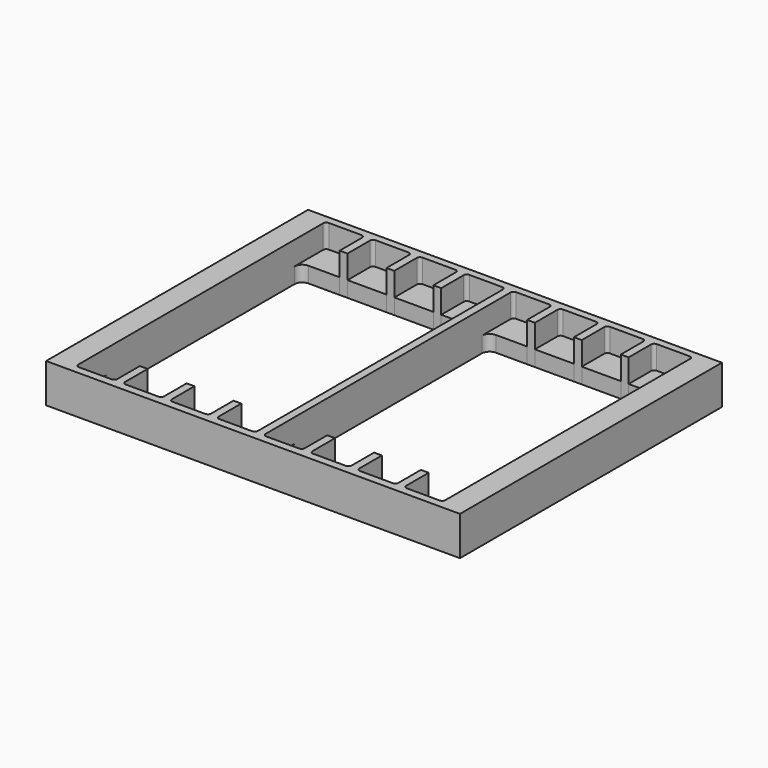
from build123d import *

# Parameters (mm, degrees)
F3_DEPTH = 10
F4_DEPTH = 10
F6_DEPTH = 25
F7_DEPTH = 25
F8_DEPTH = 25


# Not quite as in the source:
# - a feature names something its author has since deleted; it is built from what else it names


with BuildPart() as f3:
    # F0 (on Top) → F3 (new body)
    with BuildSketch(Plane.XY):
        Polygon((0, 104.6779751778), (-132.5, 104.6779751778), (-132.5, -105), (0, -105), (132.5, -105), (132.5, 104.6779751778), align=None)
        with BuildLine():
            Line((-57.5, -80), (-62.5, -80))
            Line((-62.5, -80), (-62.5, -98))
            ThreePointArc((-62.5, -98), (-63.0857864376, -99.4142135624), (-64.5, -100))
            Line((-64.5, -100), (-85.5, -100))
            ThreePointArc((-85.5, -100), (-86.9142135624, -99.4142135624), (-87.5, -98))
            Line((-87.5, -98), (-87.5, -80))
            Line((-87.5, -80), (-92.5, -80))
            Line((-92.5, -80), (-92.5, -98))
            ThreePointArc((-92.5, -98), (-93.0857864376, -99.4142135624), (-94.5, -100))
            Line((-94.5, -100), (-115.5, -100))
            ThreePointArc((-115.5, -100), (-116.9142135624, -99.4142135624), (-117.5, -98))
            Line((-117.5, -98), (-117.5, -75))
            Line((-117.5, -75), (-117.5, 75))
            Line((-117.5, 75), (-117.5, 98))
            ThreePointArc((-117.5, 98), (-116.9142135624, 99.4142135624), (-115.5, 100))
            Line((-115.5, 100), (-94.5, 100))
            ThreePointArc((-94.5, 100), (-93.0857864376, 99.4142135624), (-92.5, 98))
            Line((-92.5, 98), (-92.5, 80))
            Line((-92.5, 80), (-87.5, 80))
            Line((-87.5, 80), (-87.5, 98))
            ThreePointArc((-87.5, 98), (-86.9142135624, 99.4142135624), (-85.5, 100))
            Line((-85.5, 100), (-64.5, 100))
            ThreePointArc((-64.5, 100), (-63.0857864376, 99.4142135624), (-62.5, 98))
            Line((-62.5, 98), (-62.5, 80))
            Line((-62.5, 80), (-57.5, 80))
            Line((-57.5, 80), (-57.5, 98))
            ThreePointArc((-57.5, 98), (-56.9142135624, 99.4142135624), (-55.5, 100))
            Line((-55.5, 100), (-34.5, 100))
            ThreePointArc((-34.5, 100), (-33.0857864376, 99.4142135624), (-32.5, 98))
            Line((-32.5, 98), (-32.5, 80))
            Line((-32.5, 80), (-27.5, 80))
            Line((-27.5, 80), (-27.5, 98))
            ThreePointArc((-27.5, 98), (-26.9142135624, 99.4142135624), (-25.5, 100))
            Line((-25.5, 100), (-4.5, 100))
            ThreePointArc((-4.5, 100), (-3.0857864376, 99.4142135624), (-2.5, 98))
            Line((-2.5, 98), (-2.5, 75))
            Line((-2.5, 75), (-2.5, -75))
            Line((-2.5, -75), (-2.5, -98))
            ThreePointArc((-2.5, -98), (-3.0857864376, -99.4142135624), (-4.5, -100))
            Line((-4.5, -100), (-25.5, -100))
            ThreePointArc((-25.5, -100), (-26.9142135624, -99.4142135624), (-27.5, -98))
            Line((-27.5, -98), (-27.5, -80))
            Line((-27.5, -80), (-32.5, -80))
            Line((-32.5, -80), (-32.5, -98))
            ThreePointArc((-32.5, -98), (-33.0857864376, -99.4142135624), (-34.5, -100))
            Line((-34.5, -100), (-55.5, -100))
            ThreePointArc((-55.5, -100), (-56.9142135624, -99.4142135624), (-57.5, -98))
            Line((-57.5, -98), (-57.5, -80))
        make_face(mode=Mode.SUBTRACT)
        with BuildLine():
            Line((92.5, 80), (92.5, 98))
            ThreePointArc((92.5, 98), (93.0857864376, 99.4142135624), (94.5, 100))
            Line((94.5, 100), (115.5, 100))
            ThreePointArc((115.5, 100), (116.9142135624, 99.4142135624), (117.5, 98))
            Line((117.5, 98), (117.5, 75))
            Line((117.5, 75), (117.5, -75))
            Line((117.5, -75), (117.5, -98))
            ThreePointArc((117.5, -98), (116.9142135624, -99.4142135624), (115.5, -100))
            Line((115.5, -100), (94.5, -100))
            ThreePointArc((94.5, -100), (93.0857864376, -99.4142135624), (92.5, -98))
            Line((92.5, -98), (92.5, -80))
            Line((92.5, -80), (87.5, -80))
            Line((87.5, -80), (87.5, -98))
            ThreePointArc((87.5, -98), (86.9142135624, -99.4142135624), (85.5, -100))
            Line((85.5, -100), (64.5, -100))
            ThreePointArc((64.5, -100), (63.0857864376, -99.4142135624), (62.5, -98))
            Line((62.5, -98), (62.5, -80))
            Line((62.5, -80), (57.5, -80))
            Line((57.5, -80), (57.5, -98))
            ThreePointArc((57.5, -98), (56.9142135624, -99.4142135624), (55.5, -100))
            Line((55.5, -100), (34.5, -100))
            ThreePointArc((34.5, -100), (33.0857864376, -99.4142135624), (32.5, -98))
            Line((32.5, -98), (32.5, -80))
            Line((32.5, -80), (27.5, -80))
            Line((27.5, -80), (27.5, -98))
            ThreePointArc((27.5, -98), (26.9142135624, -99.4142135624), (25.5, -100))
            Line((25.5, -100), (4.5, -100))
            ThreePointArc((4.5, -100), (3.0857864376, -99.4142135624), (2.5, -98))
            Line((2.5, -98), (2.5, -75))
            Line((2.5, -75), (2.5, 75))
            Line((2.5, 75), (2.5, 98))
            ThreePointArc((2.5, 98), (3.0857864376, 99.4142135624), (4.5, 100))
            Line((4.5, 100), (25.5, 100))
            ThreePointArc((25.5, 100), (26.9142135624, 99.4142135624), (27.5, 98))
            Line((27.5, 98), (27.5, 80))
            Line((27.5, 80), (32.5, 80))
            Line((32.5, 80), (32.5, 98))
            ThreePointArc((32.5, 98), (33.0857864376, 99.4142135624), (34.5, 100))
            Line((34.5, 100), (55.5, 100))
            ThreePointArc((55.5, 100), (56.9142135624, 99.4142135624), (57.5, 98))
            Line((57.5, 98), (57.5, 80))
            Line((57.5, 80), (62.5, 80))
            Line((62.5, 80), (62.5, 98))
            ThreePointArc((62.5, 98), (63.0857864376, 99.4142135624), (64.5, 100))
            Line((64.5, 100), (85.5, 100))
            ThreePointArc((85.5, 100), (86.9142135624, 99.4142135624), (87.5, 98))
            Line((87.5, 98), (87.5, 80))
            Line((87.5, 80), (92.5, 80))
        make_face(mode=Mode.SUBTRACT)
        with BuildLine():
            ThreePointArc((-7.5, 80), (-3.9644660941, 78.5355339059), (-2.5, 75))
            Line((-2.5, 75), (-2.5, 98))
            ThreePointArc((-2.5, 98), (-3.0857864376, 99.4142135624), (-4.5, 100))
            Line((-4.5, 100), (-25.5, 100))
            ThreePointArc((-25.5, 100), (-26.9142135624, 99.4142135624), (-27.5, 98))
            Line((-27.5, 98), (-27.5, 80))
            Line((-27.5, 80), (-7.5, 80))
        make_face()
        with BuildLine():
            Line((-92.5, -98), (-92.5, -80))
            Line((-92.5, -80), (-112.5, -80))
            ThreePointArc((-112.5, -80), (-116.0355339059, -78.5355339059), (-117.5, -75))
            Line((-117.5, -75), (-117.5, -98))
            ThreePointArc((-117.5, -98), (-116.9142135624, -99.4142135624), (-115.5, -100))
            Line((-115.5, -100), (-94.5, -100))
            ThreePointArc((-94.5, -100), (-93.0857864376, -99.4142135624), (-92.5, -98))
        make_face()
        with BuildLine():
            Line((-7.5, -80), (-27.5, -80))
            Line((-27.5, -80), (-27.5, -98))
            ThreePointArc((-27.5, -98), (-26.9142135624, -99.4142135624), (-25.5, -100))
            Line((-25.5, -100), (-4.5, -100))
            ThreePointArc((-4.5, -100), (-3.0857864376, -99.4142135624), (-2.5, -98))
            Line((-2.5, -98), (-2.5, -75))
            ThreePointArc((-2.5, -75), (-3.9644660941, -78.5355339059), (-7.5, -80))
        make_face()
        with BuildLine():
            Line((-117.5, 98), (-117.5, 75))
            ThreePointArc((-117.5, 75), (-116.0355339059, 78.5355339059), (-112.5, 80))
            Line((-112.5, 80), (-92.5, 80))
            Line((-92.5, 80), (-92.5, 98))
            ThreePointArc((-92.5, 98), (-93.0857864376, 99.4142135624), (-94.5, 100))
            Line((-94.5, 100), (-115.5, 100))
            ThreePointArc((-115.5, 100), (-116.9142135624, 99.4142135624), (-117.5, 98))
        make_face()
        with BuildLine():
            Line((-87.5, 98), (-87.5, 80))
            Line((-87.5, 80), (-62.5, 80))
            Line((-62.5, 80), (-62.5, 98))
            ThreePointArc((-62.5, 98), (-63.0857864376, 99.4142135624), (-64.5, 100))
            Line((-64.5, 100), (-85.5, 100))
            ThreePointArc((-85.5, 100), (-86.9142135624, 99.4142135624), (-87.5, 98))
        make_face()
        with BuildLine():
            Line((-57.5, 80), (-32.5, 80))
            Line((-32.5, 80), (-32.5, 98))
            ThreePointArc((-32.5, 98), (-33.0857864376, 99.4142135624), (-34.5, 100))
            Line((-34.5, 100), (-55.5, 100))
            ThreePointArc((-55.5, 100), (-56.9142135624, 99.4142135624), (-57.5, 98))
            Line((-57.5, 98), (-57.5, 80))
        make_face()
        with BuildLine():
            Line((-62.5, -98), (-62.5, -80))
            Line((-62.5, -80), (-87.5, -80))
            Line((-87.5, -80), (-87.5, -98))
            ThreePointArc((-87.5, -98), (-86.9142135624, -99.4142135624), (-85.5, -100))
            Line((-85.5, -100), (-64.5, -100))
            ThreePointArc((-64.5, -100), (-63.0857864376, -99.4142135624), (-62.5, -98))
        make_face()
        with BuildLine():
            Line((-32.5, -80), (-57.5, -80))
            Line((-57.5, -80), (-57.5, -98))
            ThreePointArc((-57.5, -98), (-56.9142135624, -99.4142135624), (-55.5, -100))
            Line((-55.5, -100), (-34.5, -100))
            ThreePointArc((-34.5, -100), (-33.0857864376, -99.4142135624), (-32.5, -98))
            Line((-32.5, -98), (-32.5, -80))
        make_face()
    extrude(amount=F3_DEPTH)

    # F0 (on Top) → F4 (join)
    with BuildSketch(Plane.XY):
        with BuildLine():
            Line((7.5, 80), (27.5, 80))
            Line((27.5, 80), (27.5, 98))
            ThreePointArc((27.5, 98), (26.9142135624, 99.4142135624), (25.5, 100))
            Line((25.5, 100), (4.5, 100))
            ThreePointArc((4.5, 100), (3.0857864376, 99.4142135624), (2.5, 98))
            Line((2.5, 98), (2.5, 75))
            ThreePointArc((2.5, 75), (3.9644660941, 78.5355339059), (7.5, 80))
        make_face()
        with BuildLine():
            Line((32.5, 80), (57.5, 80))
            Line((57.5, 80), (57.5, 98))
            ThreePointArc((57.5, 98), (56.9142135624, 99.4142135624), (55.5, 100))
            Line((55.5, 100), (34.5, 100))
            ThreePointArc((34.5, 100), (33.0857864376, 99.4142135624), (32.5, 98))
            Line((32.5, 98), (32.5, 80))
        make_face()
        with BuildLine():
            Line((62.5, 80), (87.5, 80))
            Line((87.5, 80), (87.5, 98))
            ThreePointArc((87.5, 98), (86.9142135624, 99.4142135624), (85.5, 100))
            Line((85.5, 100), (64.5, 100))
            ThreePointArc((64.5, 100), (63.0857864376, 99.4142135624), (62.5, 98))
            Line((62.5, 98), (62.5, 80))
        make_face()
        with BuildLine():
            ThreePointArc((94.5, 100), (93.0857864376, 99.4142135624), (92.5, 98))
            Line((92.5, 98), (92.5, 80))
            Line((92.5, 80), (112.5, 80))
            ThreePointArc((112.5, 80), (116.0355339059, 78.5355339059), (117.5, 75))
            Line((117.5, 75), (117.5, 98))
            ThreePointArc((117.5, 98), (116.9142135624, 99.4142135624), (115.5, 100))
            Line((115.5, 100), (94.5, 100))
        make_face()
        with BuildLine():
            Line((117.5, -98), (117.5, -75))
            ThreePointArc((117.5, -75), (116.0355339059, -78.5355339059), (112.5, -80))
            Line((112.5, -80), (92.5, -80))
            Line((92.5, -80), (92.5, -98))
            ThreePointArc((92.5, -98), (93.0857864376, -99.4142135624), (94.5, -100))
            Line((94.5, -100), (115.5, -100))
            ThreePointArc((115.5, -100), (116.9142135624, -99.4142135624), (117.5, -98))
        make_face()
        with BuildLine():
            Line((87.5, -98), (87.5, -80))
            Line((87.5, -80), (62.5, -80))
            Line((62.5, -80), (62.5, -98))
            ThreePointArc((62.5, -98), (63.0857864376, -99.4142135624), (64.5, -100))
            Line((64.5, -100), (85.5, -100))
            ThreePointArc((85.5, -100), (86.9142135624, -99.4142135624), (87.5, -98))
        make_face()
        with BuildLine():
            Line((57.5, -98), (57.5, -80))
            Line((57.5, -80), (32.5, -80))
            Line((32.5, -80), (32.5, -98))
            ThreePointArc((32.5, -98), (33.0857864376, -99.4142135624), (34.5, -100))
            Line((34.5, -100), (55.5, -100))
            ThreePointArc((55.5, -100), (56.9142135624, -99.4142135624), (57.5, -98))
        make_face()
        with BuildLine():
            ThreePointArc((7.5, -80), (3.9644660941, -78.5355339059), (2.5, -75))
            Line((2.5, -75), (2.5, -98))
            ThreePointArc((2.5, -98), (3.0857864376, -99.4142135624), (4.5, -100))
            Line((4.5, -100), (25.5, -100))
            ThreePointArc((25.5, -100), (26.9142135624, -99.4142135624), (27.5, -98))
            Line((27.5, -98), (27.5, -80))
            Line((27.5, -80), (7.5, -80))
        make_face()
    extrude(amount=F4_DEPTH)


with BuildPart() as f6:
    # F0 (on Top) → F6 (new body)
    with BuildSketch(Plane.XY):
        Polygon((0, 104.6779751778), (-132.5, 104.6779751778), (-132.5, -105), (0, -105), (132.5, -105), (132.5, 104.6779751778), align=None)
        with BuildLine():
            Line((-57.5, -80), (-62.5, -80))
            Line((-62.5, -80), (-62.5, -98))
            ThreePointArc((-62.5, -98), (-63.0857864376, -99.4142135624), (-64.5, -100))
            Line((-64.5, -100), (-85.5, -100))
            ThreePointArc((-85.5, -100), (-86.9142135624, -99.4142135624), (-87.5, -98))
            Line((-87.5, -98), (-87.5, -80))
            Line((-87.5, -80), (-92.5, -80))
            Line((-92.5, -80), (-92.5, -98))
            ThreePointArc((-92.5, -98), (-93.0857864376, -99.4142135624), (-94.5, -100))
            Line((-94.5, -100), (-115.5, -100))
            ThreePointArc((-115.5, -100), (-116.9142135624, -99.4142135624), (-117.5, -98))
            Line((-117.5, -98), (-117.5, -75))
            Line((-117.5, -75), (-117.5, 75))
            Line((-117.5, 75), (-117.5, 98))
            ThreePointArc((-117.5, 98), (-116.9142135624, 99.4142135624), (-115.5, 100))
            Line((-115.5, 100), (-94.5, 100))
            ThreePointArc((-94.5, 100), (-93.0857864376, 99.4142135624), (-92.5, 98))
            Line((-92.5, 98), (-92.5, 80))
            Line((-92.5, 80), (-87.5, 80))
            Line((-87.5, 80), (-87.5, 98))
            ThreePointArc((-87.5, 98), (-86.9142135624, 99.4142135624), (-85.5, 100))
            Line((-85.5, 100), (-64.5, 100))
            ThreePointArc((-64.5, 100), (-63.0857864376, 99.4142135624), (-62.5, 98))
            Line((-62.5, 98), (-62.5, 80))
            Line((-62.5, 80), (-57.5, 80))
            Line((-57.5, 80), (-57.5, 98))
            ThreePointArc((-57.5, 98), (-56.9142135624, 99.4142135624), (-55.5, 100))
            Line((-55.5, 100), (-34.5, 100))
            ThreePointArc((-34.5, 100), (-33.0857864376, 99.4142135624), (-32.5, 98))
            Line((-32.5, 98), (-32.5, 80))
            Line((-32.5, 80), (-27.5, 80))
            Line((-27.5, 80), (-27.5, 98))
            ThreePointArc((-27.5, 98), (-26.9142135624, 99.4142135624), (-25.5, 100))
            Line((-25.5, 100), (-4.5, 100))
            ThreePointArc((-4.5, 100), (-3.0857864376, 99.4142135624), (-2.5, 98))
            Line((-2.5, 98), (-2.5, 75))
            Line((-2.5, 75), (-2.5, -75))
            Line((-2.5, -75), (-2.5, -98))
            ThreePointArc((-2.5, -98), (-3.0857864376, -99.4142135624), (-4.5, -100))
            Line((-4.5, -100), (-25.5, -100))
            ThreePointArc((-25.5, -100), (-26.9142135624, -99.4142135624), (-27.5, -98))
            Line((-27.5, -98), (-27.5, -80))
            Line((-27.5, -80), (-32.5, -80))
            Line((-32.5, -80), (-32.5, -98))
            ThreePointArc((-32.5, -98), (-33.0857864376, -99.4142135624), (-34.5, -100))
            Line((-34.5, -100), (-55.5, -100))
            ThreePointArc((-55.5, -100), (-56.9142135624, -99.4142135624), (-57.5, -98))
            Line((-57.5, -98), (-57.5, -80))
        make_face(mode=Mode.SUBTRACT)
        with BuildLine():
            Line((92.5, 80), (92.5, 98))
            ThreePointArc((92.5, 98), (93.0857864376, 99.4142135624), (94.5, 100))
            Line((94.5, 100), (115.5, 100))
            ThreePointArc((115.5, 100), (116.9142135624, 99.4142135624), (117.5, 98))
            Line((117.5, 98), (117.5, 75))
            Line((117.5, 75), (117.5, -75))
            Line((117.5, -75), (117.5, -98))
            ThreePointArc((117.5, -98), (116.9142135624, -99.4142135624), (115.5, -100))
            Line((115.5, -100), (94.5, -100))
            ThreePointArc((94.5, -100), (93.0857864376, -99.4142135624), (92.5, -98))
            Line((92.5, -98), (92.5, -80))
            Line((92.5, -80), (87.5, -80))
            Line((87.5, -80), (87.5, -98))
            ThreePointArc((87.5, -98), (86.9142135624, -99.4142135624), (85.5, -100))
            Line((85.5, -100), (64.5, -100))
            ThreePointArc((64.5, -100), (63.0857864376, -99.4142135624), (62.5, -98))
            Line((62.5, -98), (62.5, -80))
            Line((62.5, -80), (57.5, -80))
            Line((57.5, -80), (57.5, -98))
            ThreePointArc((57.5, -98), (56.9142135624, -99.4142135624), (55.5, -100))
            Line((55.5, -100), (34.5, -100))
            ThreePointArc((34.5, -100), (33.0857864376, -99.4142135624), (32.5, -98))
            Line((32.5, -98), (32.5, -80))
            Line((32.5, -80), (27.5, -80))
            Line((27.5, -80), (27.5, -98))
            ThreePointArc((27.5, -98), (26.9142135624, -99.4142135624), (25.5, -100))
            Line((25.5, -100), (4.5, -100))
            ThreePointArc((4.5, -100), (3.0857864376, -99.4142135624), (2.5, -98))
            Line((2.5, -98), (2.5, -75))
            Line((2.5, -75), (2.5, 75))
            Line((2.5, 75), (2.5, 98))
            ThreePointArc((2.5, 98), (3.0857864376, 99.4142135624), (4.5, 100))
            Line((4.5, 100), (25.5, 100))
            ThreePointArc((25.5, 100), (26.9142135624, 99.4142135624), (27.5, 98))
            Line((27.5, 98), (27.5, 80))
            Line((27.5, 80), (32.5, 80))
            Line((32.5, 80), (32.5, 98))
            ThreePointArc((32.5, 98), (33.0857864376, 99.4142135624), (34.5, 100))
            Line((34.5, 100), (55.5, 100))
            ThreePointArc((55.5, 100), (56.9142135624, 99.4142135624), (57.5, 98))
            Line((57.5, 98), (57.5, 80))
            Line((57.5, 80), (62.5, 80))
            Line((62.5, 80), (62.5, 98))
            ThreePointArc((62.5, 98), (63.0857864376, 99.4142135624), (64.5, 100))
            Line((64.5, 100), (85.5, 100))
            ThreePointArc((85.5, 100), (86.9142135624, 99.4142135624), (87.5, 98))
            Line((87.5, 98), (87.5, 80))
            Line((87.5, 80), (92.5, 80))
        make_face(mode=Mode.SUBTRACT)
    extrude(amount=F6_DEPTH)


with BuildPart() as f7:
    # F0 (on Top) → F7 (new body)
    with BuildSketch(Plane.XY):
        Polygon((0, 104.6779751778), (-132.5, 104.6779751778), (-132.5, -105), (0, -105), (132.5, -105), (132.5, 104.6779751778), align=None)
        with BuildLine():
            Line((-57.5, -80), (-62.5, -80))
            Line((-62.5, -80), (-62.5, -98))
            ThreePointArc((-62.5, -98), (-63.0857864376, -99.4142135624), (-64.5, -100))
            Line((-64.5, -100), (-85.5, -100))
            ThreePointArc((-85.5, -100), (-86.9142135624, -99.4142135624), (-87.5, -98))
            Line((-87.5, -98), (-87.5, -80))
            Line((-87.5, -80), (-92.5, -80))
            Line((-92.5, -80), (-92.5, -98))
            ThreePointArc((-92.5, -98), (-93.0857864376, -99.4142135624), (-94.5, -100))
            Line((-94.5, -100), (-115.5, -100))
            ThreePointArc((-115.5, -100), (-116.9142135624, -99.4142135624), (-117.5, -98))
            Line((-117.5, -98), (-117.5, -75))
            Line((-117.5, -75), (-117.5, 75))
            Line((-117.5, 75), (-117.5, 98))
            ThreePointArc((-117.5, 98), (-116.9142135624, 99.4142135624), (-115.5, 100))
            Line((-115.5, 100), (-94.5, 100))
            ThreePointArc((-94.5, 100), (-93.0857864376, 99.4142135624), (-92.5, 98))
            Line((-92.5, 98), (-92.5, 80))
            Line((-92.5, 80), (-87.5, 80))
            Line((-87.5, 80), (-87.5, 98))
            ThreePointArc((-87.5, 98), (-86.9142135624, 99.4142135624), (-85.5, 100))
            Line((-85.5, 100), (-64.5, 100))
            ThreePointArc((-64.5, 100), (-63.0857864376, 99.4142135624), (-62.5, 98))
            Line((-62.5, 98), (-62.5, 80))
            Line((-62.5, 80), (-57.5, 80))
            Line((-57.5, 80), (-57.5, 98))
            ThreePointArc((-57.5, 98), (-56.9142135624, 99.4142135624), (-55.5, 100))
            Line((-55.5, 100), (-34.5, 100))
            ThreePointArc((-34.5, 100), (-33.0857864376, 99.4142135624), (-32.5, 98))
            Line((-32.5, 98), (-32.5, 80))
            Line((-32.5, 80), (-27.5, 80))
            Line((-27.5, 80), (-27.5, 98))
            ThreePointArc((-27.5, 98), (-26.9142135624, 99.4142135624), (-25.5, 100))
            Line((-25.5, 100), (-4.5, 100))
            ThreePointArc((-4.5, 100), (-3.0857864376, 99.4142135624), (-2.5, 98))
            Line((-2.5, 98), (-2.5, 75))
            Line((-2.5, 75), (-2.5, -75))
            Line((-2.5, -75), (-2.5, -98))
            ThreePointArc((-2.5, -98), (-3.0857864376, -99.4142135624), (-4.5, -100))
            Line((-4.5, -100), (-25.5, -100))
            ThreePointArc((-25.5, -100), (-26.9142135624, -99.4142135624), (-27.5, -98))
            Line((-27.5, -98), (-27.5, -80))
            Line((-27.5, -80), (-32.5, -80))
            Line((-32.5, -80), (-32.5, -98))
            ThreePointArc((-32.5, -98), (-33.0857864376, -99.4142135624), (-34.5, -100))
            Line((-34.5, -100), (-55.5, -100))
            ThreePointArc((-55.5, -100), (-56.9142135624, -99.4142135624), (-57.5, -98))
            Line((-57.5, -98), (-57.5, -80))
        make_face(mode=Mode.SUBTRACT)
        with BuildLine():
            Line((92.5, 80), (92.5, 98))
            ThreePointArc((92.5, 98), (93.0857864376, 99.4142135624), (94.5, 100))
            Line((94.5, 100), (115.5, 100))
            ThreePointArc((115.5, 100), (116.9142135624, 99.4142135624), (117.5, 98))
            Line((117.5, 98), (117.5, 75))
            Line((117.5, 75), (117.5, -75))
            Line((117.5, -75), (117.5, -98))
            ThreePointArc((117.5, -98), (116.9142135624, -99.4142135624), (115.5, -100))
            Line((115.5, -100), (94.5, -100))
            ThreePointArc((94.5, -100), (93.0857864376, -99.4142135624), (92.5, -98))
            Line((92.5, -98), (92.5, -80))
            Line((92.5, -80), (87.5, -80))
            Line((87.5, -80), (87.5, -98))
            ThreePointArc((87.5, -98), (86.9142135624, -99.4142135624), (85.5, -100))
            Line((85.5, -100), (64.5, -100))
            ThreePointArc((64.5, -100), (63.0857864376, -99.4142135624), (62.5, -98))
            Line((62.5, -98), (62.5, -80))
            Line((62.5, -80), (57.5, -80))
            Line((57.5, -80), (57.5, -98))
            ThreePointArc((57.5, -98), (56.9142135624, -99.4142135624), (55.5, -100))
            Line((55.5, -100), (34.5, -100))
            ThreePointArc((34.5, -100), (33.0857864376, -99.4142135624), (32.5, -98))
            Line((32.5, -98), (32.5, -80))
            Line((32.5, -80), (27.5, -80))
            Line((27.5, -80), (27.5, -98))
            ThreePointArc((27.5, -98), (26.9142135624, -99.4142135624), (25.5, -100))
            Line((25.5, -100), (4.5, -100))
            ThreePointArc((4.5, -100), (3.0857864376, -99.4142135624), (2.5, -98))
            Line((2.5, -98), (2.5, -75))
            Line((2.5, -75), (2.5, 75))
            Line((2.5, 75), (2.5, 98))
            ThreePointArc((2.5, 98), (3.0857864376, 99.4142135624), (4.5, 100))
            Line((4.5, 100), (25.5, 100))
            ThreePointArc((25.5, 100), (26.9142135624, 99.4142135624), (27.5, 98))
            Line((27.5, 98), (27.5, 80))
            Line((27.5, 80), (32.5, 80))
            Line((32.5, 80), (32.5, 98))
            ThreePointArc((32.5, 98), (33.0857864376, 99.4142135624), (34.5, 100))
            Line((34.5, 100), (55.5, 100))
            ThreePointArc((55.5, 100), (56.9142135624, 99.4142135624), (57.5, 98))
            Line((57.5, 98), (57.5, 80))
            Line((57.5, 80), (62.5, 80))
            Line((62.5, 80), (62.5, 98))
            ThreePointArc((62.5, 98), (63.0857864376, 99.4142135624), (64.5, 100))
            Line((64.5, 100), (85.5, 100))
            ThreePointArc((85.5, 100), (86.9142135624, 99.4142135624), (87.5, 98))
            Line((87.5, 98), (87.5, 80))
            Line((87.5, 80), (92.5, 80))
        make_face(mode=Mode.SUBTRACT)
    extrude(amount=F7_DEPTH)


with BuildPart() as f8:
    # F0 (on Top) → F8 (new body)
    with BuildSketch(Plane.XY):
        Polygon((0, 104.6779751778), (-132.5, 104.6779751778), (-132.5, -105), (0, -105), (132.5, -105), (132.5, 104.6779751778), align=None)
        with BuildLine():
            Line((-57.5, -80), (-62.5, -80))
            Line((-62.5, -80), (-62.5, -98))
            ThreePointArc((-62.5, -98), (-63.0857864376, -99.4142135624), (-64.5, -100))
            Line((-64.5, -100), (-85.5, -100))
            ThreePointArc((-85.5, -100), (-86.9142135624, -99.4142135624), (-87.5, -98))
            Line((-87.5, -98), (-87.5, -80))
            Line((-87.5, -80), (-92.5, -80))
            Line((-92.5, -80), (-92.5, -98))
            ThreePointArc((-92.5, -98), (-93.0857864376, -99.4142135624), (-94.5, -100))
            Line((-94.5, -100), (-115.5, -100))
            ThreePointArc((-115.5, -100), (-116.9142135624, -99.4142135624), (-117.5, -98))
            Line((-117.5, -98), (-117.5, -75))
            Line((-117.5, -75), (-117.5, 75))
            Line((-117.5, 75), (-117.5, 98))
            ThreePointArc((-117.5, 98), (-116.9142135624, 99.4142135624), (-115.5, 100))
            Line((-115.5, 100), (-94.5, 100))
            ThreePointArc((-94.5, 100), (-93.0857864376, 99.4142135624), (-92.5, 98))
            Line((-92.5, 98), (-92.5, 80))
            Line((-92.5, 80), (-87.5, 80))
            Line((-87.5, 80), (-87.5, 98))
            ThreePointArc((-87.5, 98), (-86.9142135624, 99.4142135624), (-85.5, 100))
            Line((-85.5, 100), (-64.5, 100))
            ThreePointArc((-64.5, 100), (-63.0857864376, 99.4142135624), (-62.5, 98))
            Line((-62.5, 98), (-62.5, 80))
            Line((-62.5, 80), (-57.5, 80))
            Line((-57.5, 80), (-57.5, 98))
            ThreePointArc((-57.5, 98), (-56.9142135624, 99.4142135624), (-55.5, 100))
            Line((-55.5, 100), (-34.5, 100))
            ThreePointArc((-34.5, 100), (-33.0857864376, 99.4142135624), (-32.5, 98))
            Line((-32.5, 98), (-32.5, 80))
            Line((-32.5, 80), (-27.5, 80))
            Line((-27.5, 80), (-27.5, 98))
            ThreePointArc((-27.5, 98), (-26.9142135624, 99.4142135624), (-25.5, 100))
            Line((-25.5, 100), (-4.5, 100))
            ThreePointArc((-4.5, 100), (-3.0857864376, 99.4142135624), (-2.5, 98))
            Line((-2.5, 98), (-2.5, 75))
            Line((-2.5, 75), (-2.5, -75))
            Line((-2.5, -75), (-2.5, -98))
            ThreePointArc((-2.5, -98), (-3.0857864376, -99.4142135624), (-4.5, -100))
            Line((-4.5, -100), (-25.5, -100))
            ThreePointArc((-25.5, -100), (-26.9142135624, -99.4142135624), (-27.5, -98))
            Line((-27.5, -98), (-27.5, -80))
            Line((-27.5, -80), (-32.5, -80))
            Line((-32.5, -80), (-32.5, -98))
            ThreePointArc((-32.5, -98), (-33.0857864376, -99.4142135624), (-34.5, -100))
            Line((-34.5, -100), (-55.5, -100))
            ThreePointArc((-55.5, -100), (-56.9142135624, -99.4142135624), (-57.5, -98))
            Line((-57.5, -98), (-57.5, -80))
        make_face(mode=Mode.SUBTRACT)
        with BuildLine():
            Line((92.5, 80), (92.5, 98))
            ThreePointArc((92.5, 98), (93.0857864376, 99.4142135624), (94.5, 100))
            Line((94.5, 100), (115.5, 100))
            ThreePointArc((115.5, 100), (116.9142135624, 99.4142135624), (117.5, 98))
            Line((117.5, 98), (117.5, 75))
            Line((117.5, 75), (117.5, -75))
            Line((117.5, -75), (117.5, -98))
            ThreePointArc((117.5, -98), (116.9142135624, -99.4142135624), (115.5, -100))
            Line((115.5, -100), (94.5, -100))
            ThreePointArc((94.5, -100), (93.0857864376, -99.4142135624), (92.5, -98))
            Line((92.5, -98), (92.5, -80))
            Line((92.5, -80), (87.5, -80))
            Line((87.5, -80), (87.5, -98))
            ThreePointArc((87.5, -98), (86.9142135624, -99.4142135624), (85.5, -100))
            Line((85.5, -100), (64.5, -100))
            ThreePointArc((64.5, -100), (63.0857864376, -99.4142135624), (62.5, -98))
            Line((62.5, -98), (62.5, -80))
            Line((62.5, -80), (57.5, -80))
            Line((57.5, -80), (57.5, -98))
            ThreePointArc((57.5, -98), (56.9142135624, -99.4142135624), (55.5, -100))
            Line((55.5, -100), (34.5, -100))
            ThreePointArc((34.5, -100), (33.0857864376, -99.4142135624), (32.5, -98))
            Line((32.5, -98), (32.5, -80))
            Line((32.5, -80), (27.5, -80))
            Line((27.5, -80), (27.5, -98))
            ThreePointArc((27.5, -98), (26.9142135624, -99.4142135624), (25.5, -100))
            Line((25.5, -100), (4.5, -100))
            ThreePointArc((4.5, -100), (3.0857864376, -99.4142135624), (2.5, -98))
            Line((2.5, -98), (2.5, -75))
            Line((2.5, -75), (2.5, 75))
            Line((2.5, 75), (2.5, 98))
            ThreePointArc((2.5, 98), (3.0857864376, 99.4142135624), (4.5, 100))
            Line((4.5, 100), (25.5, 100))
            ThreePointArc((25.5, 100), (26.9142135624, 99.4142135624), (27.5, 98))
            Line((27.5, 98), (27.5, 80))
            Line((27.5, 80), (32.5, 80))
            Line((32.5, 80), (32.5, 98))
            ThreePointArc((32.5, 98), (33.0857864376, 99.4142135624), (34.5, 100))
            Line((34.5, 100), (55.5, 100))
            ThreePointArc((55.5, 100), (56.9142135624, 99.4142135624), (57.5, 98))
            Line((57.5, 98), (57.5, 80))
            Line((57.5, 80), (62.5, 80))
            Line((62.5, 80), (62.5, 98))
            ThreePointArc((62.5, 98), (63.0857864376, 99.4142135624), (64.5, 100))
            Line((64.5, 100), (85.5, 100))
            ThreePointArc((85.5, 100), (86.9142135624, 99.4142135624), (87.5, 98))
            Line((87.5, 98), (87.5, 80))
            Line((87.5, 80), (92.5, 80))
        make_face(mode=Mode.SUBTRACT)
    extrude(amount=F8_DEPTH)


solid = Compound([f3.part, f6.part, f7.part, f8.part])
